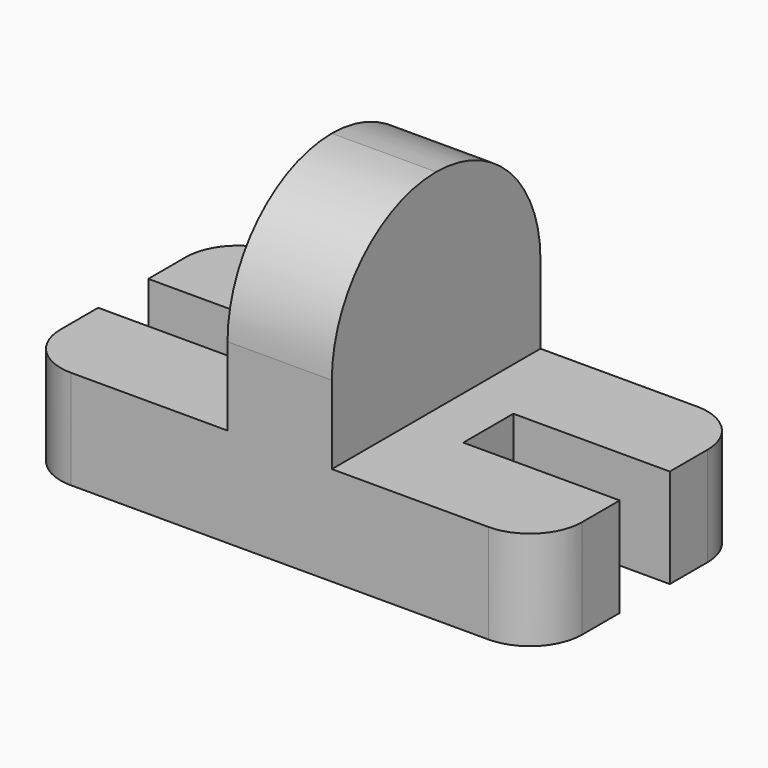
from build123d import *

# Parameters (mm, degrees)
F1_DEPTH = 48.26
F3_DEPTH = 101.6
F4_R     = 63.49999
F5_R     = 25.4


# Not quite as in the source:
# - a fillet or chamfer is up to 0.001 mm smaller than in the source, because OpenCascade refuses the exact size
# - a feature names something its author has since deleted; it is built from what else it names


with BuildPart() as f1:
    # F0 (on Top) → F1 (new body)
    with BuildSketch(Plane.XY):
        Polygon((-254, 0), (0, 0), (0, 48.26), (-76.2, 48.26), (-76.2, 78.74), (0, 78.74), (0, 127), (-101.6, 127), (-152.4, 127), (-254, 127), (-254, 78.74), (-177.8, 78.74), (-177.8, 48.26), (-254, 48.26), align=None)
    extrude(amount=F1_DEPTH)

    # F2 (on face) → F3 (join)
    with BuildSketch(Plane.XY.offset(48.26)):
        Polygon((-101.6, 127), (-127, 127), (-152.4, 127), (-152.4, 0), (-101.6, 0), align=None)
    extrude(amount=F3_DEPTH)

    # F4 (radius 63.5 in the source; OpenCascade refuses exactly that, so slightly less here)
    f4_edges = [f1.edges().sort_by_distance(p)[0] for p in [
        (-127, 0, 149.86),
        (-127, 127, 149.86),
    ]]
    fillet(f4_edges, radius=F4_R)

    # F5
    f5_edges = [f1.edges().sort_by_distance(p)[0] for p in [
        (-254, 0, 24.13),
        (0, 0, 24.13),
        (-254, 127, 24.13),
        (0, 127, 24.13),
    ]]
    fillet(f5_edges, radius=F5_R)


solid = f1.part
